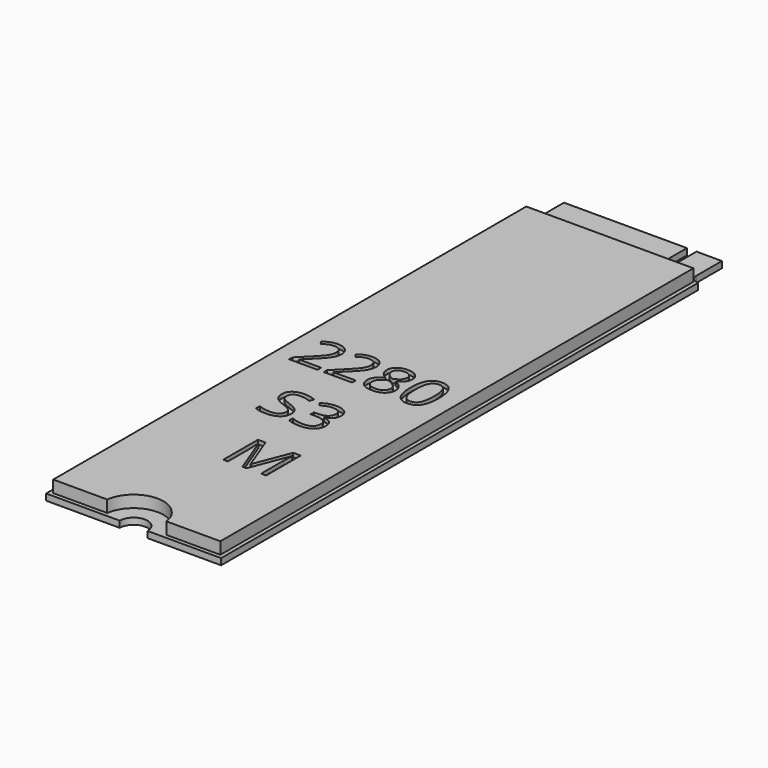
from build123d import *

# Parameters (mm, degrees)
F2_W          = 22
F2_H          = 80
F3_DEPTH      = 0.8
F4_W          = 21
F4_H          = 74.3
F5_DEPTH      = 1.5
F7_DEPTH      = 0.801
F8_R          = 1.75
F9_DEPTH      = 2.301
F11_DEPTH     = 1.5
F12_TEXT_SIZE = 7.6075757129
F13_DEPTH     = 0.5


# Not quite as in the source:
# - Text() gives the source's letters only with a copy of the font that has no kerning and outlines rounded to 1/6400 em; it was checked with that copy


with BuildPart() as f3:
    # F2 (on Top) → F3 (new body)
    with BuildSketch(Plane.XY):
        Rectangle(F2_W, F2_H)
    extrude(amount=F3_DEPTH)

    # F4 (on face) → F5 (join)
    with BuildSketch(Plane.XY.offset(0.8)):
        with Locations((0, -2.35)):
            Rectangle(F4_W, F4_H)
    extrude(amount=F5_DEPTH)

    # F6 (on face) → F7 (cut, through all)
    with BuildSketch(Plane.XY.offset(0.8)):
        with BuildLine():
            Line((-9.925, 36), (-9.925, 40))
            Line((-9.925, 40), (-11, 40))
            Line((-11, 40), (-11, 34.925))
            ThreePointArc((-11, 34.925), (-10.2398602102, 35.2398602102), (-9.925, 36))
        make_face()
        with BuildLine():
            Line((11, 40), (9.925, 40))
            Line((9.925, 40), (9.925, 36))
            ThreePointArc((9.925, 36), (10.2398602102, 35.2398602102), (11, 34.925))
            Line((11, 34.925), (11, 40))
        make_face()
        with BuildLine():
            Line((5.53, 40), (5.53, 36.6))
            ThreePointArc((5.53, 36.6), (6.13, 36), (6.73, 36.6))
            Line((6.73, 36.6), (6.73, 40))
            Line((6.73, 40), (5.53, 40))
        make_face()
    extrude(amount=-F7_DEPTH, mode=Mode.SUBTRACT)

    # F8 (on face) → F9 (cut, through all)
    with BuildSketch(Plane(origin=(0, 0, 0), x_dir=(1, 0, 0), z_dir=(0, 0, -1))):
        with Locations((0, 40)):
            Circle(F8_R)
    extrude(amount=-F9_DEPTH, mode=Mode.SUBTRACT)

    # F10 (on face) → F11 (cut, through all)
    with BuildSketch(Plane.XY.offset(2.3)):
        with BuildLine():
            ThreePointArc((-1.6770509831, -39.5), (0, -38.25), (1.6770509831, -39.5))
            Line((1.6770509831, -39.5), (3.7165171868, -39.5))
            ThreePointArc((3.7165171868, -39.5), (0, -36.25), (-3.7165171868, -39.5))
            Line((-3.7165171868, -39.5), (-1.6770509831, -39.5))
        make_face()
    extrude(amount=-F11_DEPTH, mode=Mode.SUBTRACT)

    # F12 (on face) → F13 (cut)
    with BuildSketch(Plane.XY.offset(2.3)):
        with Locations((-8.756438514, -5.0887272567)):
            Text('2280', F12_TEXT_SIZE, font='Open Sans', text_align=(TextAlign.LEFT, TextAlign.BOTTOM))
        with Locations((-4.8028765106, -15.4350302262)):
            Text('S3', F12_TEXT_SIZE, font='Open Sans', text_align=(TextAlign.LEFT, TextAlign.BOTTOM))
        with Locations((-0.8493145073, -25.7813331958)):
            Text('M', F12_TEXT_SIZE, font='Open Sans', text_align=(TextAlign.LEFT, TextAlign.BOTTOM))
    extrude(amount=-F13_DEPTH, mode=Mode.SUBTRACT)


solid = f3.part
